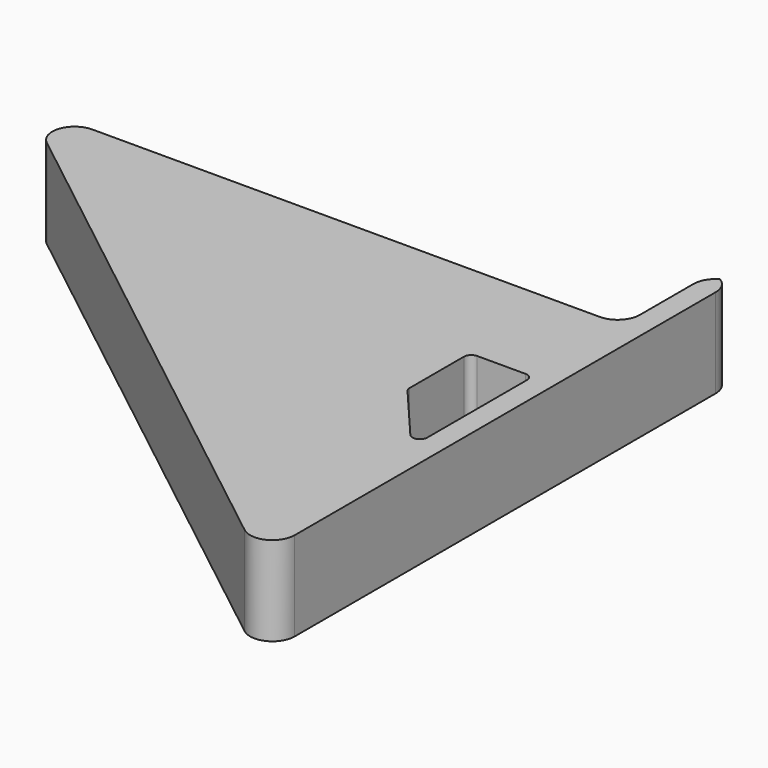
from build123d import *

# Parameters (mm, degrees)
F1_DEPTH    = 12
F3_DEPTH    = 9
F4_R        = 1.5
F5_DEPTH    = 4
F6_T1_DEPTH = 12
F6_T3_DEPTH = 9
F6_T5_DEPTH = 9
F6_T7_DEPTH = 12
F7_R        = 1


# Not quite as in the source:
# - a fillet or chamfer that OpenCascade refuses, or shapes differently, is made with other operations: its cross-section is extruded or revolved along the edge and cut away or added


with BuildPart() as f1:
    # F0 (on Top) → F1 (new body)
    with BuildSketch(Plane.XY):
        Polygon((-83, 65), (0, 0), (0, 80), (-3, 80), (-3, 65), align=None)
        Polygon((-11.5, 50), (-3, 50), (-3, 29.5), (-11.5, 39.5), align=None, mode=Mode.SUBTRACT)
    extrude(amount=F1_DEPTH)

    # F2 (on face) → F3 (cut)
    with BuildSketch(Plane.XY.offset(12)):
        Polygon((-4, 54), (-4, 61), (-71.4047410676, 61), (-4, 8.2131545856), (-4, 24.5002801184), (-15.5, 38.0296918831), (-15.5, 54), align=None)
    extrude(amount=-F3_DEPTH, mode=Mode.SUBTRACT)

    # F4 (on face) → F5 (cut)
    with BuildSketch(Plane(origin=(0, 65, 0), x_dir=(-1, 0, 0), z_dir=(0, 1, 0))):
        with Locations((50, 7.5)):
            Circle(F4_R)
        with Locations((25, 7.5)):
            Circle(F4_R)
    extrude(amount=-F5_DEPTH, mode=Mode.SUBTRACT)

    # F6: fillet of radius 3 on 12 edges, made by hand

    # F6_s2 → F6_t1 (join)
    with BuildSketch(Plane.XY):
        with BuildLine():
            ThreePointArc((-6, 65), (-3.8786796564, 65.8786796564), (-3, 68))
            Line((-3, 68), (-2.94, 68))
            Line((-2.94, 68), (-2.94, 64.94))
            Line((-2.94, 64.94), (-6, 64.94))
            Line((-6, 64.94), (-6, 65))
        make_face()
    extrude(amount=F6_T1_DEPTH)

    # F6_s4 → F6_t3 (join)
    with BuildSketch(Plane.XY.offset(3)):
        with BuildLine():
            ThreePointArc((-4, 57), (-4.8786796564, 54.8786796564), (-7, 54))
            Line((-7, 54), (-7, 53.94))
            Line((-7, 53.94), (-3.94, 53.94))
            Line((-3.94, 53.94), (-3.94, 57))
            Line((-3.94, 57), (-4, 57))
        make_face()
        with BuildLine():
            ThreePointArc((-4, 58), (-4.8786796564, 60.1213203436), (-7, 61))
            Line((-7, 61), (-7, 61.06))
            Line((-7, 61.06), (-3.94, 61.06))
            Line((-3.94, 61.06), (-3.94, 58))
            Line((-3.94, 58), (-4, 58))
        make_face()
        with BuildLine():
            ThreePointArc((-4, 23.3975490307), (-4.1842004812, 24.4325722527), (-4.7141820467, 25.340494291))
            Line((-4.7141820467, 25.340494291), (-4.6684656877, 25.3793531962))
            Line((-4.6684656877, 25.3793531962), (-3.94, 24.5223347402))
            Line((-3.94, 24.5223347402), (-3.94, 23.3975490307))
            Line((-3.94, 23.3975490307), (-4, 23.3975490307))
        make_face()
        with BuildLine():
            ThreePointArc((-8.8496919869, 12.0111061416), (-5.6864315702, 11.6758853817), (-4, 14.3730205248))
            Line((-4, 14.3730205248), (-3.94, 14.3730205248))
            Line((-3.94, 14.3730205248), (-3.94, 8.2131545856))
            Line((-3.94, 8.2131545856), (-4.0369938397, 8.165916298))
            Line((-4.0369938397, 8.165916298), (-8.8866858266, 11.9638678539))
            Line((-8.8866858266, 11.9638678539), (-8.8496919869, 12.0111061416))
        make_face()
        with BuildLine():
            ThreePointArc((-62.7082968683, 61), (-65.544292562, 58.9783294052), (-64.5579888552, 55.6380856168))
            Line((-64.5579888552, 55.6380856168), (-64.5949826949, 55.5908473291))
            Line((-64.5949826949, 55.5908473291), (-71.4417349073, 60.9527617123))
            Line((-71.4417349073, 60.9527617123), (-71.4047410676, 61.06))
            Line((-71.4047410676, 61.06), (-62.7082968683, 61.06))
            Line((-62.7082968683, 61.06), (-62.7082968683, 61))
        make_face()
    extrude(amount=F6_T3_DEPTH)

    # F6_s6 → F6_t5 (cut)
    with BuildSketch(Plane.XY.offset(3)):
        with BuildLine():
            ThreePointArc((-15.5, 51), (-14.6213203436, 53.1213203436), (-12.5, 54))
            Line((-12.5, 54), (-12.5, 54.06))
            Line((-12.5, 54.06), (-15.56, 54.06))
            Line((-15.56, 54.06), (-15.56, 51))
            Line((-15.56, 51), (-15.5, 51))
        make_face()
        with BuildLine():
            ThreePointArc((-14.7858179533, 37.1894777105), (-15.3157995188, 38.0973997488), (-15.5, 39.1324229708))
            Line((-15.5, 39.1324229708), (-15.56, 39.1324229708))
            Line((-15.56, 39.1324229708), (-15.56, 38.0076372613))
            Line((-15.56, 38.0076372613), (-14.8315343123, 37.1506188053))
            Line((-14.8315343123, 37.1506188053), (-14.7858179533, 37.1894777105))
        make_face()
    extrude(amount=F6_T5_DEPTH, mode=Mode.SUBTRACT)

    # F6_s8 → F6_t7 (cut)
    with BuildSketch(Plane.XY):
        with BuildLine():
            ThreePointArc((-76.1532477876, 59.6380856168), (-77.1395514944, 62.9783294052), (-74.3035558007, 65))
            Line((-74.3035558007, 65), (-74.3035558007, 65.06))
            Line((-74.3035558007, 65.06), (-83, 65.06))
            Line((-83, 65.06), (-83.0369938397, 64.9527617123))
            Line((-83.0369938397, 64.9527617123), (-76.1902416273, 59.5908473291))
            Line((-76.1902416273, 59.5908473291), (-76.1532477876, 59.6380856168))
        make_face()
        with BuildLine():
            ThreePointArc((0, 80), (-2.1213203436, 79.1213203436), (-3, 77))
            Line((-3, 77), (-3.06, 77))
            Line((-3.06, 77), (-3.06, 80.06))
            Line((-3.06, 80.06), (0, 80.06))
            Line((0, 80.06), (0, 80))
        make_face()
        with BuildLine():
            ThreePointArc((-4.8496919869, 3.797951556), (-1.6864315702, 3.4627307961), (0, 6.1598659392))
            Line((0, 6.1598659392), (0.06, 6.1598659392))
            Line((0.06, 6.1598659392), (0.06, 0))
            Line((0.06, 0), (-0.0369938397, -0.0472382877))
            Line((-0.0369938397, -0.0472382877), (-4.8866858266, 3.7507132683))
            Line((-4.8866858266, 3.7507132683), (-4.8496919869, 3.797951556))
        make_face()
        with BuildLine():
            ThreePointArc((0, 77), (-0.8786796564, 79.1213203436), (-3, 80))
            Line((-3, 80), (-3, 80.06))
            Line((-3, 80.06), (0.06, 80.06))
            Line((0.06, 80.06), (0.06, 77))
            Line((0.06, 77), (0, 77))
        make_face()
    extrude(amount=F6_T7_DEPTH, mode=Mode.SUBTRACT)

    # F7
    f7_edges = [f1.edges().sort_by_distance(p)[0] for p in [
        (-11.5, 50, 6),
        (-3, 50, 6),
        (-11.5, 39.5, 6),
        (-3, 29.5, 6),
    ]]
    fillet(f7_edges, radius=F7_R)


with BuildPart() as f8_1:
    # F8: instance of F1
    add(f1.part.mirror(Plane.XY))


solid = f8_1.part
